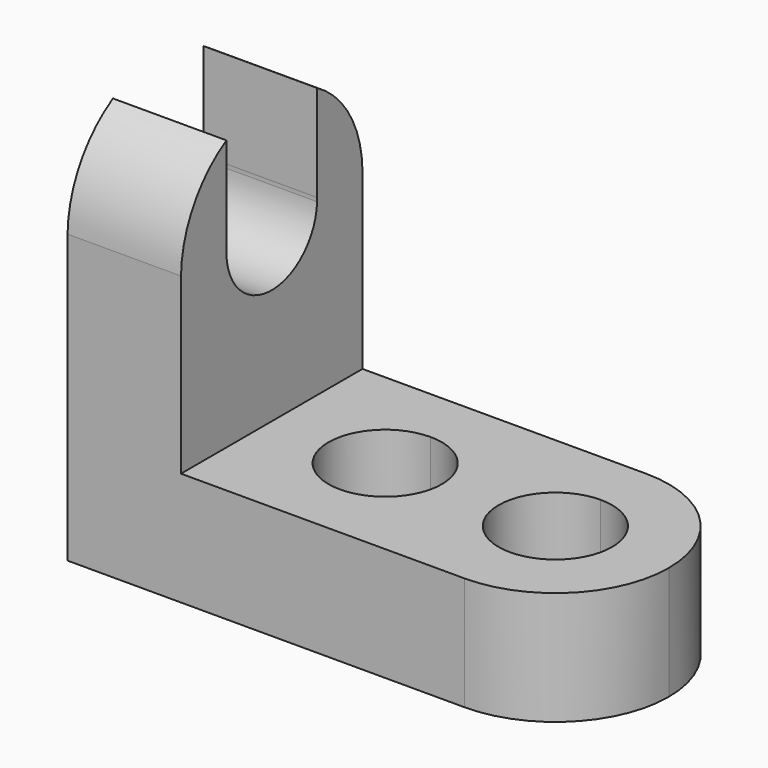
from build123d import *

# Parameters (mm, degrees)
F1_DEPTH = 25.4
F3_DEPTH = 12.701
F5_DEPTH = 12.701
F7_DEPTH = 57.151


with BuildPart() as f1:
    # F0 (on Front) → F1 (new body)
    with BuildSketch(Plane.XZ):
        Polygon((0, 44.45), (0, 0), (57.15, 0), (57.15, 12.7), (12.7, 12.7), (12.7, 44.45), align=None)
    extrude(amount=F1_DEPTH)

    # F2 (on face) → F3 (cut, through all)
    with BuildSketch(Plane.XY.offset(12.7)):
        with BuildLine():
            Line((25.4, -19.05), (25.4, -6.35))
            ThreePointArc((25.4, -6.35), (19.05, -12.7), (25.4, -19.05))
        make_face()
        with BuildLine():
            ThreePointArc((31.75, -12.7), (29.8901280605, -8.2098719395), (25.4, -6.35))
            Line((25.4, -6.35), (25.4, -19.05))
            ThreePointArc((25.4, -19.05), (29.8901280605, -17.1901280605), (31.75, -12.7))
        make_face()
        with BuildLine():
            Line((44.45, -19.05), (44.45, -6.35))
            ThreePointArc((44.45, -6.35), (38.1, -12.7), (44.45, -19.05))
        make_face()
        with BuildLine():
            ThreePointArc((50.8, -12.7), (48.9401280605, -8.2098719395), (44.45, -6.35))
            Line((44.45, -6.35), (44.45, -19.05))
            ThreePointArc((44.45, -19.05), (48.9401280605, -17.1901280605), (50.8, -12.7))
        make_face()
        with BuildLine():
            Line((57.15, 0), (44.45, 0))
            ThreePointArc((44.45, 0), (53.4302561211, -3.7197438789), (57.15, -12.7))
            Line((57.15, -12.7), (57.15, 0))
        make_face()
        with BuildLine():
            Line((57.15, -25.4), (57.15, -12.7))
            ThreePointArc((57.15, -12.7), (53.4302561211, -21.6802561211), (44.45, -25.4))
            Line((44.45, -25.4), (57.15, -25.4))
        make_face()
    extrude(amount=-F3_DEPTH, mode=Mode.SUBTRACT)

    # F4 (on face) → F5 (cut, through all)
    with BuildSketch(Plane.YZ.offset(12.7)):
        with BuildLine():
            ThreePointArc((-25.4, 32.1787146746), (-25.4018088896, 31.9643573373), (-25.4, 31.75))
            Line((-25.4, 31.75), (-25.4, 32.1787146746))
        make_face()
        with BuildLine():
            Line((0, 32.1787146746), (0, 31.75))
            ThreePointArc((0, 31.75), (0.0018088896, 31.9643573373), (0, 32.1787146746))
        make_face()
        with BuildLine():
            Line((-25.4, 44.45), (-25.4, 32.1787146746))
            ThreePointArc((-25.4, 32.1787146746), (-22.4029254465, 40.1612583888), (-15.0333830306, 44.45))
            Line((-15.0333830306, 44.45), (-25.4, 44.45))
        make_face()
        with BuildLine():
            ThreePointArc((-10.3666169694, 44.45), (-2.9970745535, 40.1612583888), (0, 32.1787146746))
            Line((0, 32.1787146746), (0, 44.45))
            Line((0, 44.45), (-10.3666169694, 44.45))
        make_face()
    extrude(amount=-F5_DEPTH, mode=Mode.SUBTRACT)

    # F6 (on face) → F7 (cut, through all)
    with BuildSketch(Plane(origin=(0, 0, 0), x_dir=(0, -1, 0), z_dir=(-1, 0, 0))):
        with BuildLine():
            Line((6.3536190682, 32.1787146746), (6.3536190682, 31.75))
            Line((6.3536190682, 31.75), (19.0463809318, 31.75))
            Line((19.0463809318, 31.75), (19.0463809318, 32.1787146746))
            ThreePointArc((19.0463809318, 32.1787146746), (12.7, 38.3143573373), (6.3536190682, 32.1787146746))
        make_face()
        with BuildLine():
            Line((19.0463809318, 31.75), (6.3536190682, 31.75))
            ThreePointArc((6.3536190682, 31.75), (12.7, 25.6143573373), (19.0463809318, 31.75))
        make_face()
        with BuildLine():
            ThreePointArc((6.3536190682, 32.1787146746), (6.35, 31.9643573373), (6.3536190682, 31.75))
            Line((6.3536190682, 31.75), (6.3536190682, 32.1787146746))
        make_face()
        with BuildLine():
            Line((19.0463809318, 32.1787146746), (19.0463809318, 31.75))
            ThreePointArc((19.0463809318, 31.75), (19.0490951685, 31.8571633942), (19.05, 31.9643573373))
            ThreePointArc((19.05, 31.9643573373), (19.0490951685, 32.0715512803), (19.0463809318, 32.1787146746))
        make_face()
        with BuildLine():
            Line((6.3536190682, 42.9670569213), (6.3536190682, 32.1787146746))
            ThreePointArc((6.3536190682, 32.1787146746), (12.7, 38.3143573373), (19.0463809318, 32.1787146746))
            Line((19.0463809318, 32.1787146746), (19.0463809318, 42.9670569213))
            ThreePointArc((19.0463809318, 42.9670569213), (17.1027668181, 43.8787013567), (15.0333830306, 44.45))
            Line((15.0333830306, 44.45), (10.3666169694, 44.45))
            ThreePointArc((10.3666169694, 44.45), (8.2972331819, 43.8787013567), (6.3536190682, 42.9670569213))
        make_face()
    extrude(amount=-F7_DEPTH, mode=Mode.SUBTRACT)


solid = f1.part
